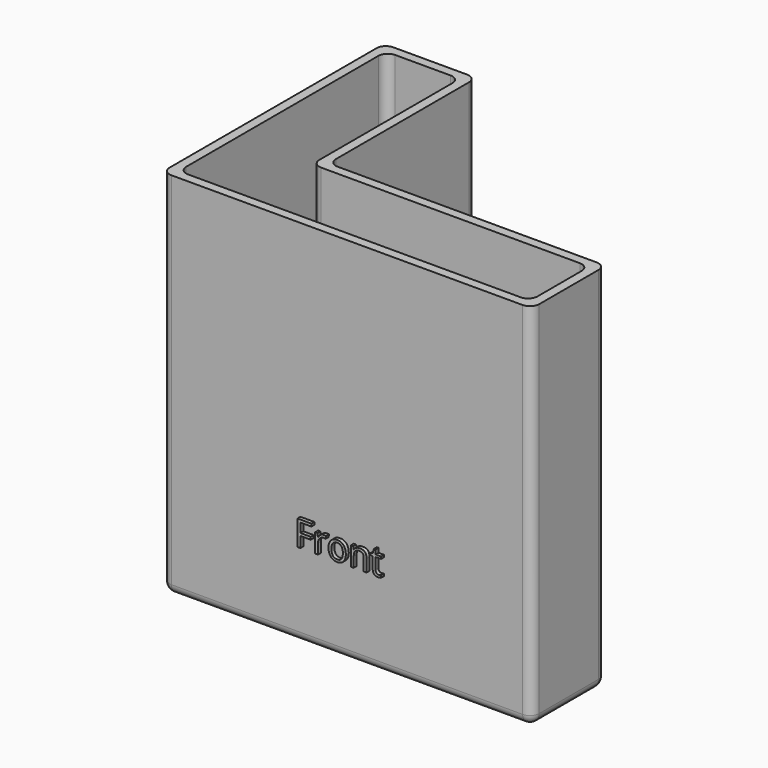
from build123d import *

# Parameters (mm, degrees)
F1_DEPTH     = 20
F3_DEPTH     = 9.5
F4_R         = 0.5
F5_TEXT_SIZE = 1.9070239634
F6_DEPTH     = 0.2


# Not quite as in the source:
# - Text() gives the source's letters only with a copy of the font that has no kerning and outlines rounded to 1/6400 em; it was checked with that copy


with BuildPart() as f1:
    # F0 (on Top) → F1 (new body)
    with BuildSketch(Plane.XY):
        Polygon((-20, 0), (0, 0), (0, 5), (-15, 5), (-15, 15), (-20, 15), align=None)
    extrude(amount=F1_DEPTH)

    # F2 (on face) → F3 (cut)
    with BuildSketch(Plane.XY.offset(20)):
        Polygon((-15.5, 14.5), (-19.5, 14.5), (-19.5, 0.5), (-0.5, 0.5), (-0.5, 4.5), (-15.5, 4.5), align=None)
    extrude(amount=-F3_DEPTH, mode=Mode.SUBTRACT)

    # F4
    f4_edges = [f1.edges().sort_by_distance(p)[0] for p in [
        (-19.5, 0.5, 15.25),
        (-15, 5, 10),
        (-0.5, 0.5, 15.25),
        (-0.5, 4.5, 15.25),
        (-15.5, 4.5, 15.25),
        (-20, 0, 10),
        (-19.5, 14.5, 15.25),
        (-19.5, 7.5, 10.5),
        (-17.5, 14.5, 10.5),
        (-15.5, 14.5, 15.25),
        (-8, 4.5, 10.5),
        (-10, 0.5, 10.5),
        (0, 5, 10),
        (0, 0, 10),
        (-15, 15, 10),
        (-20, 15, 10),
        (-7.5, 5, 0),
        (-15, 10, 0),
        (0, 2.5, 0),
        (-10, 0, 0),
        (-20, 7.5, 0),
        (-17.5, 15, 0),
        (-15.5, 9.5, 10.5),
    ]]
    fillet(f4_edges, radius=F4_R)

    # F5 (on face) → F6 (join)
    with BuildSketch(Plane.XZ):
        with Locations((-12.713169679, 4.6410439536)):
            Text('Front', F5_TEXT_SIZE, font='Open Sans', text_align=(TextAlign.LEFT, TextAlign.BOTTOM))
    extrude(amount=F6_DEPTH)


solid = f1.part
